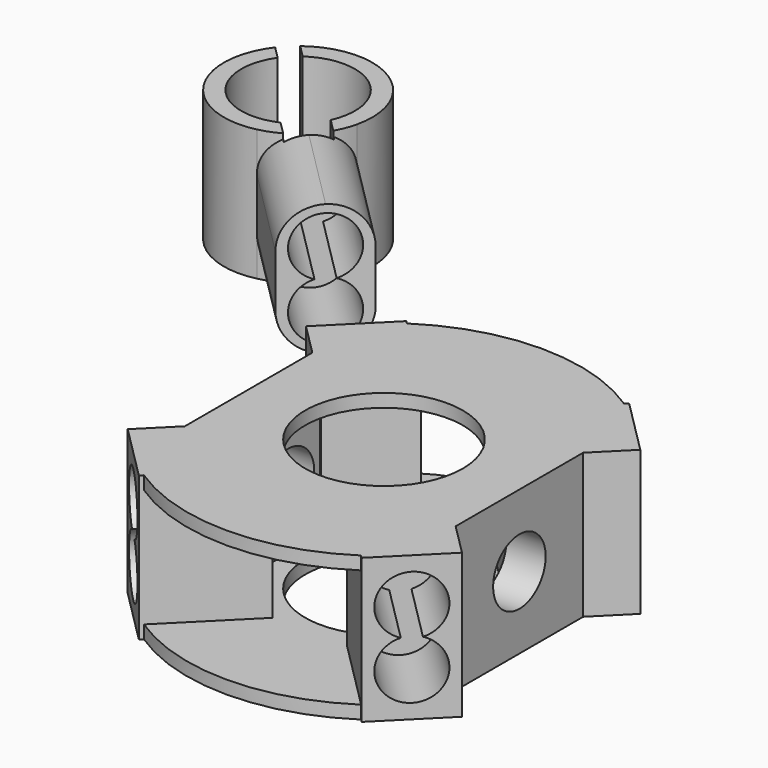
from build123d import *

# Parameters (mm, degrees)
F2_DEPTH      = 5.5
F3_R          = 15
F4_DEPTH      = 1
F5_W          = 3
F5_H          = 12.1347305831
F6_DEPTH      = 5
F7_R          = 15
F8_DEPTH      = 1
F9_R          = 6
F10_DEPTH     = 12.5
F12_DEPTH     = 100
F14_DEPTH     = 100
F15_R         = 2.5
F16_DEPTH     = 100
F17_W         = 6
F17_H         = 11
F18_DEPTH     = 1.8
F19_W         = 6
F19_H         = 9
F20_DEPTH     = 1.8
F21_W         = 6
F21_H         = 9
F22_DEPTH     = 1.8
F23_W         = 6
F23_H         = 9
F24_DEPTH     = 1.8
F25_R         = 5.65
F25_R_2       = 4.325
F26_DEPTH     = 5
F28_DEPTH     = 5
F31_R         = 5.65
F31_R_2       = 3.5
F32_DEPTH     = 0.6
F33_DEPTH     = 12.5
F35_DEPTH     = 7.338
F36_T4_DEPTH  = 25
F36_S5_R      = 5.65
F36_T6_DEPTH  = 16
F36_T10_DEPTH = 25
F36_S11_R     = 5.65
F36_T12_DEPTH = 16
F36_T16_DEPTH = 25
F36_S17_R     = 5.65
F36_T18_DEPTH = 16
F36_T22_DEPTH = 25
F36_S23_R     = 5.65
F36_T24_DEPTH = 16
F37_DEPTH     = 12.5


# Not quite as in the source:
# - a fillet or chamfer that OpenCascade refuses, or shapes differently, is made with other operations: its cross-section is extruded or revolved along the edge and cut away or added


with BuildPart() as f2:
    # F1 (on Top) → F2 (new body, symmetric)
    with BuildSketch(Plane.XY):
        Polygon((12.7279220614, 8.4852813742), (8.4852813742, 12.7279220614), (2.8284271247, 7.0710678119), (7.0710678119, 2.8284271247), align=None)
    extrude(amount=F2_DEPTH, both=True)



with BuildPart() as f2b:
    # F1 (on Top) → F2, piece 2 (new body, symmetric)
    with BuildSketch(Plane.XY):
        Polygon((8.4852813742, -12.7279220614), (12.7279220614, -8.4852813742), (7.0710678119, -2.8284271247), (2.8284271247, -7.0710678119), align=None)
    extrude(amount=F2_DEPTH, both=True)


with BuildPart() as f2c:
    # F1 (on Top) → F2, piece 3 (new body, symmetric)
    with BuildSketch(Plane.XY):
        Polygon((-8.4852813742, -12.7279220614), (-2.8284271247, -7.0710678119), (-7.0710678119, -2.8284271247), (-12.7279220614, -8.4852813742), align=None)
    extrude(amount=F2_DEPTH, both=True)


with BuildPart() as f2d:
    # F1 (on Top) → F2, piece 4 (new body, symmetric)
    with BuildSketch(Plane.XY):
        Polygon((-2.8284271247, 7.0710678119), (-8.4852813742, 12.7279220614), (-12.7279220614, 8.4852813742), (-7.0710678119, 2.8284271247), align=None)
    extrude(amount=F2_DEPTH, both=True)


with BuildPart() as f2_1:
    add(f2.part)

    add(f2b.part)  # F4 merges F2b

    add(f2c.part)  # F4 merges F2c

    add(f2d.part)  # F4 merges F2d
    # F3 (on face) → F4 (join)
    with BuildSketch(Plane.XY.offset(5.5)):
        Circle(F3_R)
    extrude(amount=-F4_DEPTH)

    # F5 (on Top) → F6 (join, symmetric)
    with BuildSketch(Plane.XY):
        with Locations((-8.8100059787, 0)):
            Rectangle(F5_W, F5_H)
        with Locations((8.8100059787, 0)):
            Rectangle(F5_W, F5_H)
    extrude(amount=F6_DEPTH, both=True)

    # F7 (on face) → F8 (join)
    with BuildSketch(Plane(origin=(0, 0, -5.5), x_dir=(1, 0, 0), z_dir=(0, 0, -1))):
        Circle(F7_R)
    extrude(amount=-F8_DEPTH)

    # F9 (on Top) → F10 (cut, symmetric)
    with BuildSketch(Plane.XY):
        Circle(F9_R)
    extrude(amount=F10_DEPTH, both=True, mode=Mode.SUBTRACT)

    # F11 (on face) → F12 (cut)
    with BuildSketch(Plane(origin=(10.6066017178, 10.6066017178, 0), x_dir=(-0.7071067812, 0.7071067812, 0), z_dir=(0.7071067812, 0.7071067812, 0))):
        with BuildLine():
            ThreePointArc((-0.6633249581, 0), (0, -4.4), (0.6633249581, 0))
            ThreePointArc((0.6633249581, 0), (0, 4.4), (-0.6633249581, 0))
        make_face()
    extrude(amount=-F12_DEPTH, mode=Mode.SUBTRACT)

    # F13 (on face) → F14 (cut)
    with BuildSketch(Plane(origin=(-10.6066017178, 10.6066017178, 0), x_dir=(-0.7071067812, -0.7071067812, 0), z_dir=(-0.7071067812, 0.7071067812, 0))):
        with BuildLine():
            ThreePointArc((-0.6633249581, 0), (0, -4.4), (0.6633249581, 0))
            ThreePointArc((0.6633249581, 0), (0, 4.4), (-0.6633249581, 0))
        make_face()
    extrude(amount=-F14_DEPTH, mode=Mode.SUBTRACT)

    # F15 (on face) → F16 (cut)
    with BuildSketch(Plane(origin=(-10.3100059787, 0, 0), x_dir=(0, -1, 0), z_dir=(-1, 0, 0))):
        Circle(F15_R)
    extrude(amount=-F16_DEPTH, mode=Mode.SUBTRACT)

    # F17 (on face) → F18 (join)
    with BuildSketch(Plane(origin=(4.9497474683, -4.9497474683, 0), x_dir=(-0.7071067812, -0.7071067812, 0), z_dir=(-0.7071067812, 0.7071067812, 0))):
        Rectangle(F17_W, F17_H)
    extrude(amount=-F18_DEPTH)

    # F19 (on face) → F20 (join)
    with BuildSketch(Plane(origin=(-4.9497474683, 4.9497474683, 0), x_dir=(0.7071067812, 0.7071067812, 0), z_dir=(0.7071067812, -0.7071067812, 0))):
        Rectangle(F19_W, F19_H)
    extrude(amount=-F20_DEPTH)

    # F21 (on face) → F22 (join)
    with BuildSketch(Plane(origin=(-4.9497474683, -4.9497474683, 0), x_dir=(-0.7071067812, 0.7071067812, 0), z_dir=(0.7071067812, 0.7071067812, 0))):
        Rectangle(F21_W, F21_H)
    extrude(amount=-F22_DEPTH)

    # F23 (on face) → F24 (join)
    with BuildSketch(Plane(origin=(4.9497474683, 4.9497474683, 0), x_dir=(0.7071067812, -0.7071067812, 0), z_dir=(-0.7071067812, -0.7071067812, 0))):
        Rectangle(F23_W, F23_H)
    extrude(amount=-F24_DEPTH)

    # F37 (cut, symmetric): faces of the model
    f37_faces = [f2_1.faces().sort_by_distance(p)[0] for p in [
        (-12.4284977083, 0, -4.5),
        (12.4284977083, 0, -4.5),
    ]]
    extrude(f37_faces, amount=F37_DEPTH, both=True, mode=Mode.SUBTRACT)


with BuildPart() as f26:
    # F25 (on Top) → F26 (new body, symmetric)
    with BuildSketch(Plane.XY):
        with Locations((-32.7036886299, 32.7036886299)):
            Circle(F25_R)
        with Locations((-32.7036886299, 32.7036886299)):
            Circle(F25_R_2, mode=Mode.SUBTRACT)
    extrude(amount=F26_DEPTH, both=True)

    # F27 (on Top) → F28 (join, symmetric)
    with BuildSketch(Plane.XY):
        Polygon((-27.1969214916, 31.4395621787), (-31.4395621787, 27.1969214916), (-24.3684943668, 20.1258536797), (-20.1258536797, 24.3684943668), align=None)
    extrude(amount=F28_DEPTH, both=True)

    # F31 (on face) → F32 (join)
    with BuildSketch(Plane(origin=(0, 0, -5), x_dir=(1, 0, 0), z_dir=(0, 0, -1))):
        with Locations((-32.7036886299, -32.7036886299)):
            Circle(F31_R)
        with Locations((-32.7036886299, -32.7036886299)):
            Circle(F31_R_2, mode=Mode.SUBTRACT)
    extrude(amount=-F32_DEPTH)

    # F30 (on Top) + F29 (on Top) → F33 (cut, symmetric)
    with BuildSketch(Plane.XY):
        Polygon((-38.2369231114, 37.1762629396), (-35.653056475, 34.5923963032), (-34.5923963032, 35.653056475), (-37.1762629396, 38.2369231114), align=None)
    with BuildSketch(Plane.XY):
        Polygon((-29.6454518012, 31.7667721448), (-31.7667721448, 29.6454518012), (-29.6454518012, 27.5241314577), (-27.5241314577, 29.6454518012), align=None)
    extrude(amount=F33_DEPTH, both=True, mode=Mode.SUBTRACT)

    # F34 (on face) → F35 (cut)
    with BuildSketch(Plane(origin=(-22.2471740233, 22.2471740233, 0), x_dir=(0.7071067812, 0.7071067812, 0), z_dir=(0.7071067812, -0.7071067812, 0))):
        with BuildLine():
            ThreePointArc((-0.6633249581, 0), (0, -4.4), (0.6633249581, 0))
            ThreePointArc((0.6633249581, 0), (0, 4.4), (-0.6633249581, 0))
        make_face()
    extrude(amount=-F35_DEPTH, mode=Mode.SUBTRACT)

    # F36: fillet of radius 3 on 4 edges, made by hand


with BuildPart() as f36_tool2:
    # F36_s3 → F36_t4 (new body)
    with BuildSketch(Plane(origin=(-16.9438731644, 16.9438731644, 0), x_dir=(0, 0, 1), z_dir=(-0.7071067812, 0.7071067812, 0))):
        with BuildLine():
            ThreePointArc((5, 0), (4.1213203436, 2.1213203436), (2, 3))
            Line((2, 3), (5, 3))
            Line((5, 3), (5, 0))
        make_face()
    extrude(amount=F36_T4_DEPTH)

    # F36_s5 → F36_t6 (cut, symmetric)
    with BuildSketch(Plane.XY.offset(3.5)):
        with Locations((-32.7036886299, 32.7036886299)):
            Circle(F36_S5_R)
    extrude(amount=F36_T6_DEPTH, both=True, mode=Mode.SUBTRACT)


with BuildPart() as f26_1:
    add(f26.part)

    # F36_t1: cut F36_tool2
    add(f36_tool2.part, mode=Mode.SUBTRACT)


with BuildPart() as f36_tool8:
    # F36_s9 → F36_t10 (new body)
    with BuildSketch(Plane(origin=(-34.621542694, 34.621542694, 0), x_dir=(0, 0, 1), z_dir=(0.7071067812, -0.7071067812, 0))):
        with BuildLine():
            ThreePointArc((2, 3), (4.1213203436, 2.1213203436), (5, 0))
            Line((5, 0), (5, 3))
            Line((5, 3), (2, 3))
        make_face()
    extrude(amount=F36_T10_DEPTH)

    # F36_s11 → F36_t12 (cut, symmetric)
    with BuildSketch(Plane.XY.offset(3.5)):
        with Locations((-32.7036886299, 32.7036886299)):
            Circle(F36_S11_R)
    extrude(amount=F36_T12_DEPTH, both=True, mode=Mode.SUBTRACT)


with BuildPart() as f26_2:
    add(f26_1.part)

    # F36_t7: cut F36_tool8
    add(f36_tool8.part, mode=Mode.SUBTRACT)


with BuildPart() as f36_tool14:
    # F36_s15 → F36_t16 (new body)
    with BuildSketch(Plane(origin=(-16.9438731644, 16.9438731644, 0), x_dir=(0, 0, 1), z_dir=(-0.7071067812, 0.7071067812, 0))):
        with BuildLine():
            ThreePointArc((-5, 0), (-4.1213203436, 2.1213203436), (-2, 3))
            Line((-2, 3), (-5, 3))
            Line((-5, 3), (-5, 0))
        make_face()
    extrude(amount=F36_T16_DEPTH)

    # F36_s17 → F36_t18 (cut, symmetric)
    with BuildSketch(Plane.XY.offset(-3.5)):
        with Locations((-32.7036886299, 32.7036886299)):
            Circle(F36_S17_R)
    extrude(amount=F36_T18_DEPTH, both=True, mode=Mode.SUBTRACT)


with BuildPart() as f26_3:
    add(f26_2.part)

    # F36_t13: cut F36_tool14
    add(f36_tool14.part, mode=Mode.SUBTRACT)


with BuildPart() as f36_tool20:
    # F36_s21 → F36_t22 (new body)
    with BuildSketch(Plane(origin=(-34.621542694, 34.621542694, 0), x_dir=(0, 0, 1), z_dir=(0.7071067812, -0.7071067812, 0))):
        with BuildLine():
            ThreePointArc((-2, 3), (-4.1213203436, 2.1213203436), (-5, 0))
            Line((-5, 0), (-5, 3))
            Line((-5, 3), (-2, 3))
        make_face()
    extrude(amount=F36_T22_DEPTH)

    # F36_s23 → F36_t24 (cut, symmetric)
    with BuildSketch(Plane.XY.offset(-3.5)):
        with Locations((-32.7036886299, 32.7036886299)):
            Circle(F36_S23_R)
    extrude(amount=F36_T24_DEPTH, both=True, mode=Mode.SUBTRACT)


with BuildPart() as f26_4:
    add(f26_3.part)

    # F36_t19: cut F36_tool20
    add(f36_tool20.part, mode=Mode.SUBTRACT)


solid = Compound([f2_1.part, f26_4.part])
